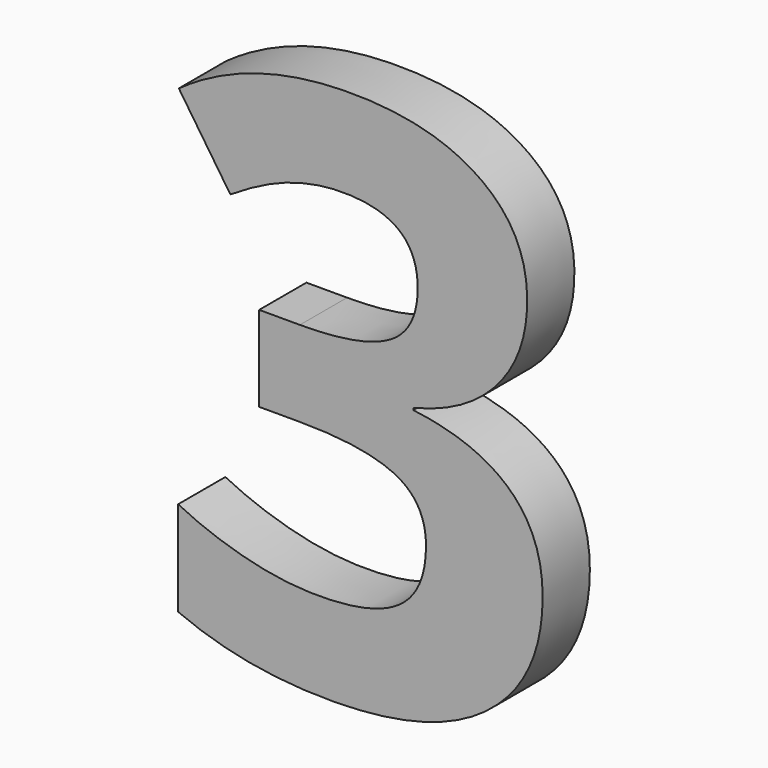
from build123d import *

# Parameters (mm, degrees)
F0_TEXT_SIZE = 62.5
F1_DEPTH     = 5


# Not quite as in the source:
# - Text() gives the source's letters only with a copy of the font that has no kerning and outlines rounded to 1/6400 em; it was checked with that copy


with BuildPart() as f1:
    # F0 (on Front) → F1 (new body)
    with BuildSketch(Plane.XZ):
        with Locations((-56.0315537701, 11.25000119)):
            Text('3', F0_TEXT_SIZE, font='Open Sans', font_style=FontStyle.BOLD, text_align=(TextAlign.LEFT, TextAlign.BOTTOM))
    extrude(amount=F1_DEPTH)


solid = f1.part
